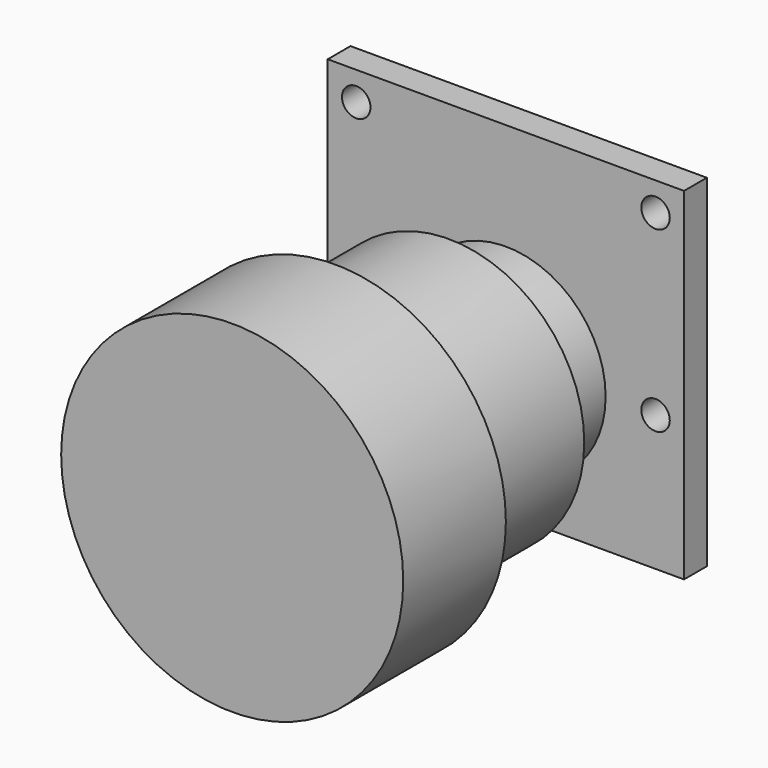
from build123d import *

# Parameters (mm, degrees)
F0_W     = 25
F0_H     = 24
F0_R     = 1
F0_R_2   = 7
F1_DEPTH = 2
F2_DEPTH = 24
F3_R     = 6
F4_DEPTH = 7
F5_START = 7
F3_R_2   = 9.5
F5_DEPTH = 10
F6_START = 17
F3_R_3   = 12
F6_DEPTH = 9


with BuildPart() as f1:
    # F0 (on Front) → F1 (new body)
    with BuildSketch(Plane.XZ):
        with Locations((0, 2.5)):
            Rectangle(F0_W, F0_H)
        with Locations((-10.5, 0)):
            Circle(F0_R, mode=Mode.SUBTRACT)
        Circle(F0_R_2, mode=Mode.SUBTRACT)
        with Locations((10.5, 0)):
            Circle(F0_R, mode=Mode.SUBTRACT)
        with Locations((-10.5, 12.5)):
            Circle(F0_R, mode=Mode.SUBTRACT)
        with Locations((10.5, 12.5)):
            Circle(F0_R, mode=Mode.SUBTRACT)
        Circle(F0_R_2)
    extrude(amount=F1_DEPTH)

    # F0 (on Front) → F2 (join)
    with BuildSketch(Plane.XZ):
        Circle(F0_R_2)
    extrude(amount=F2_DEPTH)


with BuildPart() as f4:
    # F3 (on Front) → F4 (new body)
    with BuildSketch(Plane.XZ):
        Circle(F3_R)
    extrude(amount=F4_DEPTH)

    # F3 (on Front) → F5 (join)
    with BuildSketch(Plane.XZ.offset(F5_START)):
        Circle(F3_R_2)
        Circle(F3_R, mode=Mode.SUBTRACT)
        Circle(F3_R)
    extrude(amount=F5_DEPTH)

    # F3 (on Front) → F6 (join)
    with BuildSketch(Plane.XZ.offset(F6_START)):
        Circle(F3_R_3)
        Circle(F3_R_2, mode=Mode.SUBTRACT)
        Circle(F3_R_2)
        Circle(F3_R, mode=Mode.SUBTRACT)
        Circle(F3_R)
    extrude(amount=F6_DEPTH)


solid = Compound([f1.part, f4.part])
